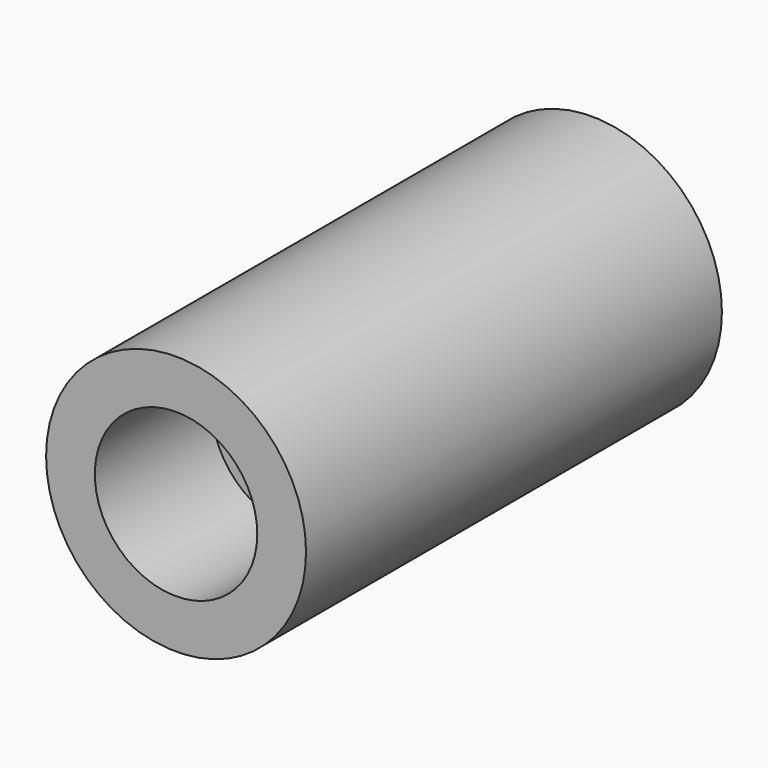
from build123d import *

# Parameters (mm, degrees)
F2_R     = 31.75
F2_R_2   = 21.59
F3_DEPTH = 44.45
F2_R_3   = 50.8
F4_DEPTH = 101.6


# Not quite as in the source:
# - a variable given as a bare number and used for a length is read in inches; the dataset says mm whatever the document's units were


with BuildPart() as f3:
    # F2 (on Front) → F3 (new body, symmetric)
    with BuildSketch(Plane.XZ):
        Circle(F2_R)
        Circle(F2_R_2, mode=Mode.SUBTRACT)
    extrude(amount=F3_DEPTH, both=True)

    # F2 (on Front) → F4 (join, symmetric)
    with BuildSketch(Plane.XZ):
        Circle(F2_R_3)
        Circle(F2_R, mode=Mode.SUBTRACT)
    extrude(amount=F4_DEPTH, both=True)


solid = f3.part
